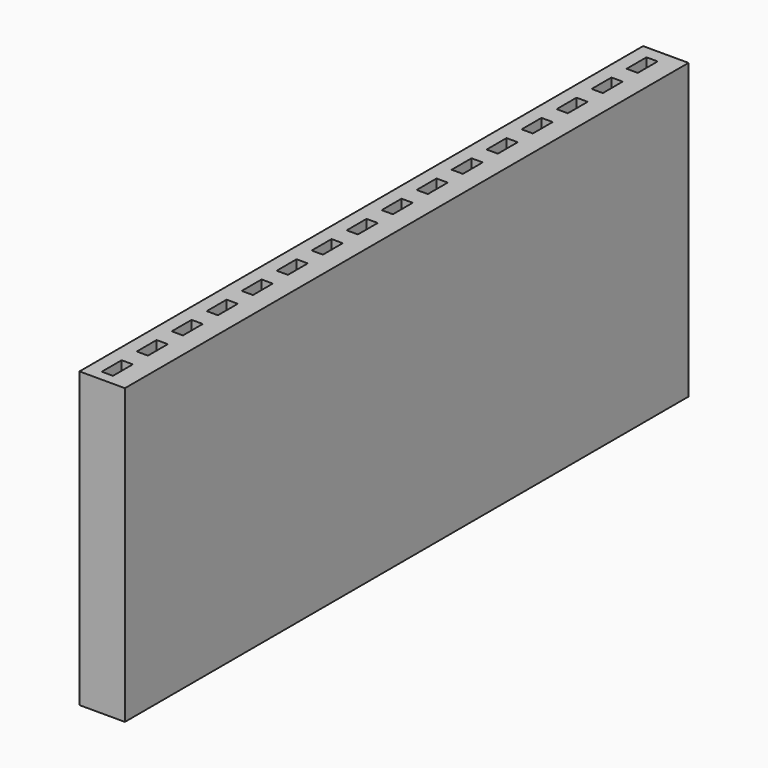
from build123d import *

# Parameters (mm, degrees)
F0_W      = 151.3
F0_H      = 48.5
F1_DEPTH  = 8
F2_W      = 1.85
F2_H      = 4.1
F3_W      = 0.25
F3_H      = 4.1
F22_DEPTH = 1.5
F23_DEPTH = 2
F24_DEPTH = 35


with BuildPart() as f1:
    # F0 (on Right) → F1 (new body)
    with BuildSketch(Plane.YZ):
        with Locations((4.7718379647, -21.296962655)):
            Rectangle(F0_W, F0_H)
    extrude(amount=F1_DEPTH)

    # F2 (on face) → F4 section 0
    with BuildSketch(Plane.XY.offset(2.953037345)):
        with Locations((1.7172626683, -67.0981232643)):
            Rectangle(F2_W, F2_H)
    # F3 (on face) → F4 section 1
    with BuildSketch(Plane(origin=(0, 0, -45.546962655), x_dir=(1, 0, 0), z_dir=(0, 0, -1))):
        with Locations((0.9037374025, 67.0926149368)):
            Rectangle(F3_W, F3_H)
    loft()

    # F3 (on face) → F5 section 0
    with BuildSketch(Plane(origin=(0, 0, -45.546962655), x_dir=(1, 0, 0), z_dir=(0, 0, -1))):
        with Locations((0.9037374025, 67.0926149368)):
            Rectangle(F3_W, F3_H)
    # F2 (on face) → F5 section 1
    with BuildSketch(Plane.XY.offset(2.953037345)):
        with Locations((1.7172626683, -67.0981232643)):
            Rectangle(F2_W, F2_H)
    loft(mode=Mode.SUBTRACT)

    # F2 (on face) → F6 section 0
    with BuildSketch(Plane.XY.offset(2.953037345)):
        with Locations((1.7172626683, -59.8781232643)):
            Rectangle(F2_W, F2_H)
    # F3 (on face) → F6 section 1
    with BuildSketch(Plane(origin=(0, 0, -45.546962655), x_dir=(1, 0, 0), z_dir=(0, 0, -1))):
        with Locations((0.9037374025, 59.8726149368)):
            Rectangle(F3_W, F3_H)
    loft(mode=Mode.SUBTRACT)

    # F2 (on face) → F7 section 0
    with BuildSketch(Plane.XY.offset(2.953037345)):
        with Locations((1.7172626683, -52.6581232643)):
            Rectangle(F2_W, F2_H)
    # F3 (on face) → F7 section 1
    with BuildSketch(Plane(origin=(0, 0, -45.546962655), x_dir=(1, 0, 0), z_dir=(0, 0, -1))):
        with Locations((0.9037374025, 52.6526149368)):
            Rectangle(F3_W, F3_H)
    loft(mode=Mode.SUBTRACT)

    # F2 (on face) → F8 section 0
    with BuildSketch(Plane.XY.offset(2.953037345)):
        with Locations((1.7172626683, -45.4381232643)):
            Rectangle(F2_W, F2_H)
    # F3 (on face) → F8 section 1
    with BuildSketch(Plane(origin=(0, 0, -45.546962655), x_dir=(1, 0, 0), z_dir=(0, 0, -1))):
        with Locations((0.9037374025, 45.4326149368)):
            Rectangle(F3_W, F3_H)
    loft(mode=Mode.SUBTRACT)

    # F3 (on face) → F9 section 0
    with BuildSketch(Plane(origin=(0, 0, -45.546962655), x_dir=(1, 0, 0), z_dir=(0, 0, -1))):
        with Locations((0.9037374025, 38.2126149368)):
            Rectangle(F3_W, F3_H)
    # F2 (on face) → F9 section 1
    with BuildSketch(Plane.XY.offset(2.953037345)):
        with Locations((1.7172626683, -38.2181232643)):
            Rectangle(F2_W, F2_H)
    loft(mode=Mode.SUBTRACT)

    # F2 (on face) → F10 section 0
    with BuildSketch(Plane.XY.offset(2.953037345)):
        with Locations((1.7172626683, -30.9981232643)):
            Rectangle(F2_W, F2_H)
    # F3 (on face) → F10 section 1
    with BuildSketch(Plane(origin=(0, 0, -45.546962655), x_dir=(1, 0, 0), z_dir=(0, 0, -1))):
        with Locations((0.9037374025, 30.9926149368)):
            Rectangle(F3_W, F3_H)
    loft(mode=Mode.SUBTRACT)

    # F3 (on face) → F11 section 0
    with BuildSketch(Plane(origin=(0, 0, -45.546962655), x_dir=(1, 0, 0), z_dir=(0, 0, -1))):
        with Locations((0.9037374025, 23.7726149368)):
            Rectangle(F3_W, F3_H)
    # F2 (on face) → F11 section 1
    with BuildSketch(Plane.XY.offset(2.953037345)):
        with Locations((1.7172626683, -23.7781232643)):
            Rectangle(F2_W, F2_H)
    loft(mode=Mode.SUBTRACT)

    # F2 (on face) → F12 section 0
    with BuildSketch(Plane.XY.offset(2.953037345)):
        with Locations((1.7172626683, -16.5581232643)):
            Rectangle(F2_W, F2_H)
    # F3 (on face) → F12 section 1
    with BuildSketch(Plane(origin=(0, 0, -45.546962655), x_dir=(1, 0, 0), z_dir=(0, 0, -1))):
        with Locations((0.9037374025, 16.5526149368)):
            Rectangle(F3_W, F3_H)
    loft()

    # F2 (on face) → F13 section 0
    with BuildSketch(Plane.XY.offset(2.953037345)):
        with Locations((1.7172626683, -16.5581232643)):
            Rectangle(F2_W, F2_H)
    # F3 (on face) → F13 section 1
    with BuildSketch(Plane(origin=(0, 0, -45.546962655), x_dir=(1, 0, 0), z_dir=(0, 0, -1))):
        with Locations((0.9037374025, 16.5526149368)):
            Rectangle(F3_W, F3_H)
    loft(mode=Mode.SUBTRACT)

    # F2 (on face) → F14 section 0
    with BuildSketch(Plane.XY.offset(2.953037345)):
        with Locations((1.7172626683, -9.3381232643)):
            Rectangle(F2_W, F2_H)
    # F3 (on face) → F14 section 1
    with BuildSketch(Plane(origin=(0, 0, -45.546962655), x_dir=(1, 0, 0), z_dir=(0, 0, -1))):
        with Locations((0.9037374025, 9.3326149368)):
            Rectangle(F3_W, F3_H)
    loft(mode=Mode.SUBTRACT)

    # F3 (on face) → F15 section 0
    with BuildSketch(Plane(origin=(0, 0, -45.546962655), x_dir=(1, 0, 0), z_dir=(0, 0, -1))):
        with Locations((0.9037374025, 2.1126149368)):
            Rectangle(F3_W, F3_H)
    # F2 (on face) → F15 section 1
    with BuildSketch(Plane.XY.offset(2.953037345)):
        with Locations((1.7172626683, -2.1181232643)):
            Rectangle(F2_W, F2_H)
    loft(mode=Mode.SUBTRACT)

    # F3 (on face) → F16 section 0
    with BuildSketch(Plane(origin=(0, 0, -45.546962655), x_dir=(1, 0, 0), z_dir=(0, 0, -1))):
        with Locations((0.9037374025, -5.1073850632)):
            Rectangle(F3_W, F3_H)
    # F2 (on face) → F16 section 1
    with BuildSketch(Plane.XY.offset(2.953037345)):
        with Locations((1.7172626683, 5.1018767357)):
            Rectangle(F2_W, F2_H)
    loft(mode=Mode.SUBTRACT)

    # F2 (on face) → F17 section 0
    with BuildSketch(Plane.XY.offset(2.953037345)):
        with Locations((1.7172626683, 12.3218767357)):
            Rectangle(F2_W, F2_H)
    # F3 (on face) → F17 section 1
    with BuildSketch(Plane(origin=(0, 0, -45.546962655), x_dir=(1, 0, 0), z_dir=(0, 0, -1))):
        with Locations((0.9037374025, -12.3273850632)):
            Rectangle(F3_W, F3_H)
    loft(mode=Mode.SUBTRACT)

    # F3 (on face) → F18 section 0
    with BuildSketch(Plane(origin=(0, 0, -45.546962655), x_dir=(1, 0, 0), z_dir=(0, 0, -1))):
        with Locations((0.9037374025, -19.5473850632)):
            Rectangle(F3_W, F3_H)
    # F2 (on face) → F18 section 1
    with BuildSketch(Plane.XY.offset(2.953037345)):
        with Locations((1.7172626683, 19.5418767357)):
            Rectangle(F2_W, F2_H)
    loft(mode=Mode.SUBTRACT)

    # F2 (on face) → F19 section 0
    with BuildSketch(Plane.XY.offset(2.953037345)):
        with Locations((1.7172626683, 26.7618767357)):
            Rectangle(F2_W, F2_H)
    # F3 (on face) → F19 section 1
    with BuildSketch(Plane(origin=(0, 0, -45.546962655), x_dir=(1, 0, 0), z_dir=(0, 0, -1))):
        with Locations((0.9037374025, -26.7673850632)):
            Rectangle(F3_W, F3_H)
    loft(mode=Mode.SUBTRACT)

    # F3 (on face) → F20 section 0
    with BuildSketch(Plane(origin=(0, 0, -45.546962655), x_dir=(1, 0, 0), z_dir=(0, 0, -1))):
        with Locations((0.9037374025, -33.9873850632)):
            Rectangle(F3_W, F3_H)
    # F2 (on face) → F20 section 1
    with BuildSketch(Plane.XY.offset(2.953037345)):
        with Locations((1.7172626683, 33.9818767357)):
            Rectangle(F2_W, F2_H)
    loft(mode=Mode.SUBTRACT)

    # F2 (on face) → F21 section 0
    with BuildSketch(Plane.XY.offset(2.953037345)):
        with Locations((1.7172626683, 41.2018767357)):
            Rectangle(F2_W, F2_H)
    # F3 (on face) → F21 section 1
    with BuildSketch(Plane(origin=(0, 0, -45.546962655), x_dir=(1, 0, 0), z_dir=(0, 0, -1))):
        with Locations((0.9037374025, -41.2073850632)):
            Rectangle(F3_W, F3_H)
    loft(mode=Mode.SUBTRACT)

    # F22 (add): a face of the model
    f22_faces = [f1.faces().sort_by_distance(p)[0] for p in [
        (0, 4.7718379647, -21.296962655),
    ]]
    extrude(f22_faces, amount=F22_DEPTH)

    # F23 (cut): a face of the model
    f23_faces = [f1.faces().sort_by_distance(p)[0] for p in [
        (8, 4.7718379647, -21.296962655),
    ]]
    extrude(f23_faces, amount=-F23_DEPTH, mode=Mode.SUBTRACT)

    # F24 (cut): a face of the model
    f24_faces = [f1.faces().sort_by_distance(p)[0] for p in [
        (2.25, 80.4218379647, -21.296962655),
    ]]
    extrude(f24_faces, amount=-F24_DEPTH, mode=Mode.SUBTRACT)


solid = f1.part
